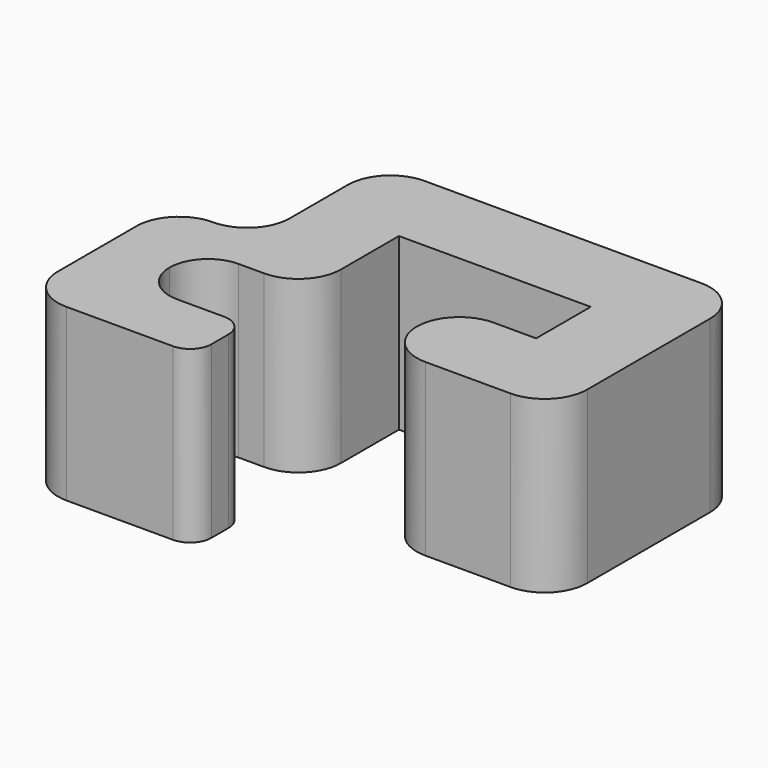
from build123d import *

# Parameters (mm, degrees)
F1_DEPTH = 4
F2_R     = 0.99999
F3_R     = 0.89999
F4_R     = 0.5


# Not quite as in the source:
# - a fillet or chamfer is up to 0.001 mm smaller than in the source, because OpenCascade refuses the exact size


with BuildPart() as f1:
    # F0 (on Top) → F1 (new body)
    with BuildSketch(Plane.XY):
        Polygon((0, -2.7), (0, 0), (4.5, 0), (4.5, -1.6), (2.5, -1.6), (2.5, -3.6), (6.5, -3.6), (6.5, 2), (-2, 2), (-2, -1.7), (-4, -1.7), (-4, -6), (0, -6), (0, -4.5), (-2.5, -4.5), (-2.5, -2.7), align=None)
    extrude(amount=F1_DEPTH)

    # F2 (radius 1 in the source; OpenCascade refuses exactly that, so slightly less here)
    f2_edges = [f1.edges().sort_by_distance(p)[0] for p in [
        (6.5, -3.6, 2),
        (6.5, 2, 2),
        (-2, 2, 2),
        (-2, -1.7, 2),
        (-4, -1.7, 2),
        (-4, -6, 2),
        (2.5, -3.6, 2),
        (0, -2.7, 2),
        (2.5, -1.6, 2),
    ]]
    fillet(f2_edges, radius=F2_R)

    # F3 (radius 0.9 in the source; OpenCascade refuses exactly that, so slightly less here)
    f3_edges = [f1.edges().sort_by_distance(p)[0] for p in [
        (-2.5, -2.7, 2),
        (-2.5, -4.5, 2),
    ]]
    fillet(f3_edges, radius=F3_R)

    # F4
    f4_edges = [f1.edges().sort_by_distance(p)[0] for p in [
        (0, -6, 2),
        (0, -4.5, 2),
    ]]
    fillet(f4_edges, radius=F4_R)


solid = f1.part
